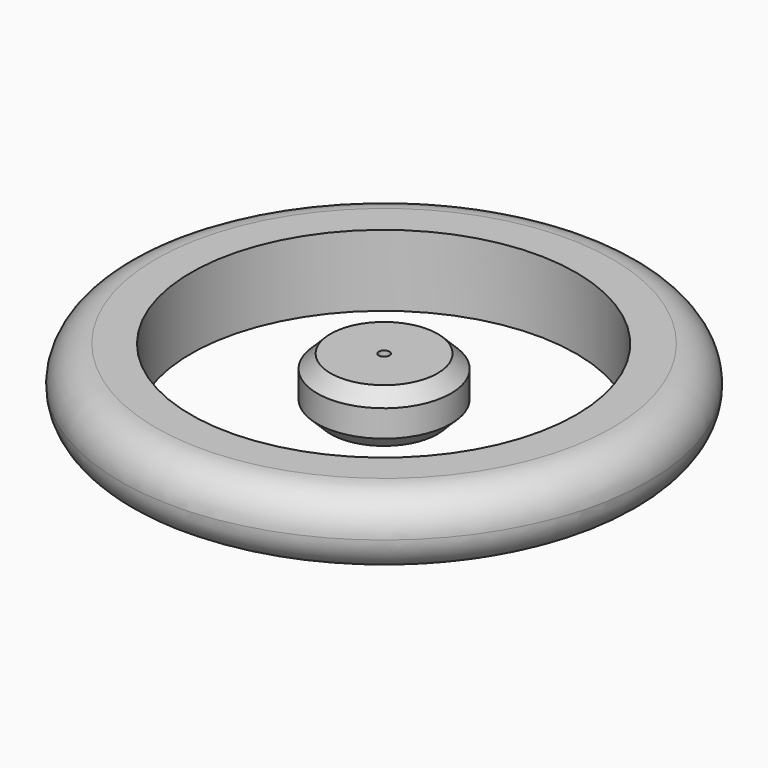
from build123d import *

# Parameters (mm, degrees)
F0_R     = 296
F0_R_2   = 216
F1_DEPTH = 80
F2_R     = 39.99999
F0_R_3   = 75
F0_R_4   = 6
F3_DEPTH = 70
F4_DEPTH = 10
F5_SIZE  = 15


# Not quite as in the source:
# - a fillet or chamfer is up to 0.001 mm smaller than in the source, because OpenCascade refuses the exact size


with BuildPart() as f1:
    # F0 (on Top) → F1 (new body)
    with BuildSketch(Plane.XY):
        Circle(F0_R)
        with Locations((0, -0.6947662914)):
            Circle(F0_R_2, mode=Mode.SUBTRACT)
    extrude(amount=-F1_DEPTH)

    # F2 (radius 40 in the source; OpenCascade refuses exactly that, so slightly less here)
    f2_edges = [f1.edges().sort_by_distance(p)[0] for p in [
        (-296, 0, 0),
        (-296, 0, -80),
    ]]
    fillet(f2_edges, radius=F2_R)


with BuildPart() as f3:
    # F0 (on Top) → F3 (new body)
    with BuildSketch(Plane.XY):
        Circle(F0_R_3)
        Circle(F0_R_4, mode=Mode.SUBTRACT)
    extrude(amount=-F3_DEPTH)

    # F4 (cut): a face of the model
    f4_faces = [f3.faces().sort_by_distance(p)[0] for p in [
        (-72.8786796564, 0, 0),
    ]]
    extrude(f4_faces, amount=-F4_DEPTH, mode=Mode.SUBTRACT)

    # F5
    f5_edges = [f3.edges().sort_by_distance(p)[0] for p in [
        (-75, 0, -10),
        (-75, 0, -70),
    ]]
    chamfer(f5_edges, length=F5_SIZE)


solid = Compound([f1.part, f3.part])
